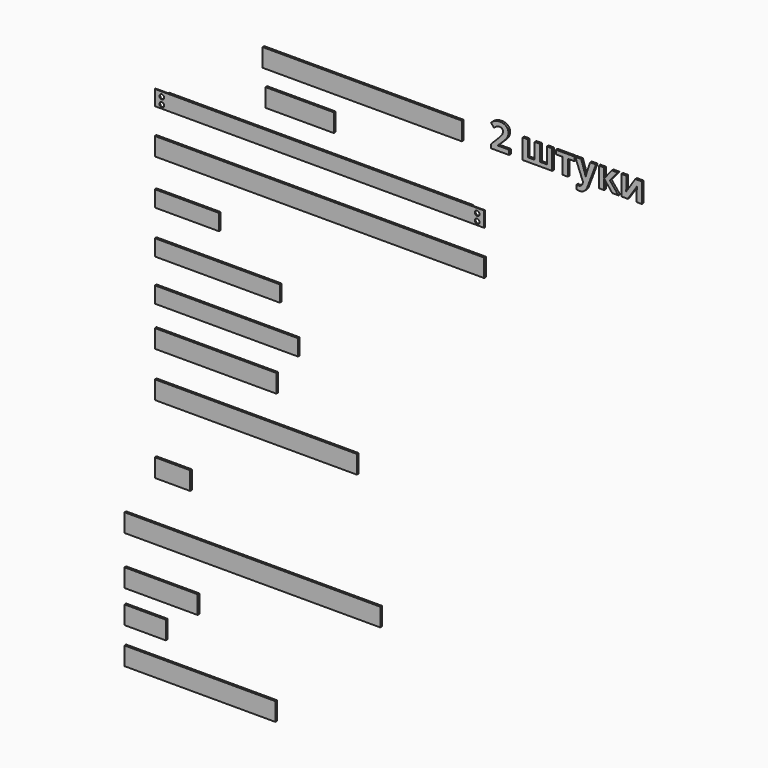
from build123d import *

# Parameters (mm, degrees)
F0_W         = 853
F0_H         = 78
F0_W_2       = 293
F0_W_3       = 54
F0_H_2       = 65
F0_R         = 10
F0_W_4       = 1302
F0_W_5       = 1410
F0_H_3       = 77
F0_W_6       = 275
F0_H_4       = 69
F0_W_7       = 535
F0_W_8       = 613
F0_W_9       = 520
F0_W_10      = 865
F0_W_11      = 151
F0_W_12      = 1095
F0_W_13      = 313
F0_W_14      = 177
F0_W_15      = 646
F0_TEXT_SIZE = 155.8384961552
F1_DEPTH     = 9
F2_DEPTH     = 5


# Not quite as in the source:
# - Text() gives the source's letters only with a copy of the font that has no kerning and outlines rounded to 1/6400 em; it was checked with that copy


with BuildPart() as f1:
    # F0 (on Front) → F1 (new body)
    with BuildSketch(Plane.XZ):
        with Locations((-362.6874928474, 57.0803574622)):
            Rectangle(F0_W, F0_H)
        with Locations((-630.4149541855, -89.7863254547)):
            Rectangle(F0_W_2, F0_H)
        with Locations((-1223.2016460896, -244.111417532)):
            Rectangle(F0_W_3, F0_H_2)
        with Locations((-1220.2016460896, -261.611417532)):
            Circle(F0_R, mode=Mode.SUBTRACT)
        with Locations((-1220.2016460896, -231.611417532)):
            Circle(F0_R, mode=Mode.SUBTRACT)
        with Locations((-545.2016460896, -244.111417532)):
            Rectangle(F0_W_4, F0_H_2)
        with Locations((132.7983539104, -244.111417532)):
            Rectangle(F0_W_3, F0_H_2)
        with Locations((129.7983539104, -261.611417532)):
            Circle(F0_R, mode=Mode.SUBTRACT)
        with Locations((129.7983539104, -231.611417532)):
            Circle(F0_R, mode=Mode.SUBTRACT)
        with Locations((-545.2016460896, -427.4489095211)):
            Rectangle(F0_W_5, F0_H_3)
        with Locations((-1112.7016460896, -624.1542129517)):
            Rectangle(F0_W_6, F0_H_4)
        with Locations((-982.7016460896, -808.6098461151)):
            Rectangle(F0_W_7, F0_H_4)
        with Locations((-943.7016460896, -986.2849740982)):
            Rectangle(F0_W_8, F0_H_4)
        with Locations((-990.2016460896, -1151.7351016998)):
            Rectangle(F0_W_9, F0_H)
        with Locations((-817.7016460896, -1344.8602304459)):
            Rectangle(F0_W_10, F0_H)
        with Locations((-1174.7016460896, -1638.410364151)):
            Rectangle(F0_W_11, F0_H)
        with Locations((-832.4077358246, -1887.9868421555)):
            Rectangle(F0_W_12, F0_H)
        with Locations((-1223.4077358246, -2095.3312263489)):
            Rectangle(F0_W_13, F0_H)
        with Locations((-1291.4077358246, -2235.2495536804)):
            Rectangle(F0_W_14, F0_H)
        with Locations((-1056.9077358246, -2389.8747310638)):
            Rectangle(F0_W_15, F0_H)
        with Locations((182.5190484524, 32.4839986861)):
            Text('2 штуки', F0_TEXT_SIZE, font='Open Sans', font_style=FontStyle.BOLD, text_align=(TextAlign.LEFT, TextAlign.BOTTOM))
    extrude(amount=F1_DEPTH)

    # F0 (on Front) → F2 (cut)
    with BuildSketch(Plane.XZ):
        with Locations((-1223.2016460896, -244.111417532)):
            Rectangle(F0_W_3, F0_H_2)
        with Locations((-1220.2016460896, -261.611417532)):
            Circle(F0_R, mode=Mode.SUBTRACT)
        with Locations((-1220.2016460896, -231.611417532)):
            Circle(F0_R, mode=Mode.SUBTRACT)
        with Locations((132.7983539104, -244.111417532)):
            Rectangle(F0_W_3, F0_H_2)
        with Locations((129.7983539104, -261.611417532)):
            Circle(F0_R, mode=Mode.SUBTRACT)
        with Locations((129.7983539104, -231.611417532)):
            Circle(F0_R, mode=Mode.SUBTRACT)
    extrude(amount=F2_DEPTH, mode=Mode.SUBTRACT)


solid = f1.part
